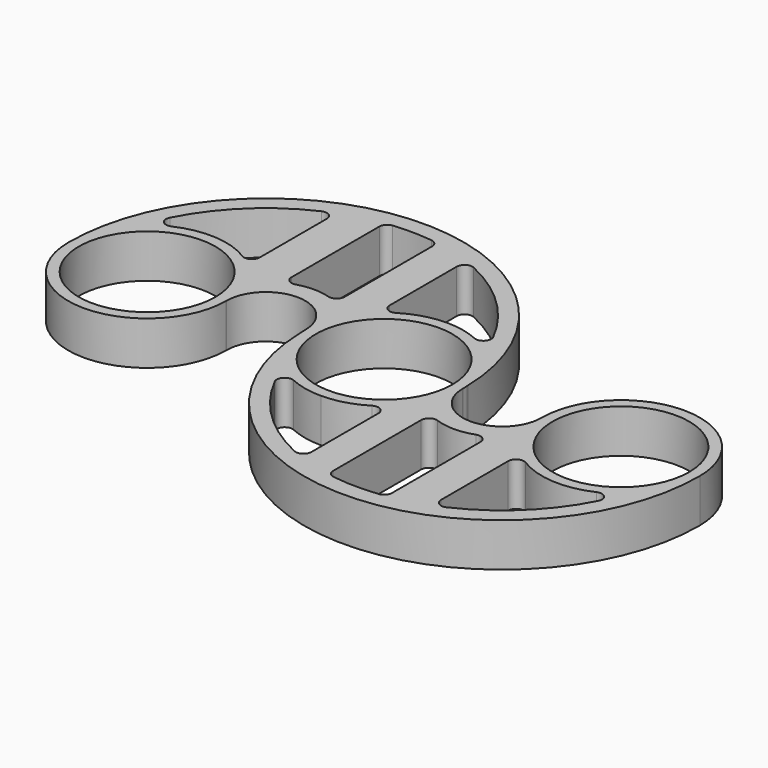
from build123d import *

# Parameters (mm, degrees)
F0_R        = 10.9855
F0_R_2      = 10.989999991
F1_DEPTH    = 7
F2_T1_DEPTH = 7
F2_T3_DEPTH = 7.1579854221
F2_T5_DEPTH = 7.1579856015
F2_T7_DEPTH = 7.1579856772
F3_R        = 1.27


# Not quite as in the source:
# - a fillet or chamfer that OpenCascade refuses, or shapes differently, is made with other operations: its cross-section is extruded or revolved along the edge and cut away or added
# - a feature names something its author has since deleted; it is built from what else it names


with BuildPart() as f1:
    # F0 (on Top) → F1 (new body)
    with BuildSketch(Plane.XY):
        with BuildLine():
            ThreePointArc((0.0122500747, -12.699994092), (8.9845861326, -8.9759240207), (12.7, 0))
            ThreePointArc((12.7, 0), (11.6341942626, 5.0926931834), (8.6156655339, 9.3306113095))
            ThreePointArc((8.6156655339, 9.3306113095), (4.6312435718, 11.8254633304), (0.0122500747, 12.699994092))
            ThreePointArc((0.0122500747, 12.699994092), (-4.6067434223, 11.8254633304), (-8.5911653844, 9.3306113095))
            ThreePointArc((-8.5911653844, 9.3306113095), (-11.6096941131, 5.0926931834), (-12.6754998505, 0))
            ThreePointArc((-12.6754998505, 0), (-11.6096941131, -5.0926931834), (-8.5911653844, -9.3306113095))
            ThreePointArc((-8.5911653844, -9.3306113095), (-4.6067434223, -11.8254633304), (0.0122500747, -12.699994092))
        make_face()
        with Locations((0.0245001495, 0)):
            Circle(F0_R, mode=Mode.SUBTRACT)
        with BuildLine():
            ThreePointArc((12.7245001495, 0), (12.716207726, 0.4588668575), (12.6913412845, 0.9171344838))
            ThreePointArc((12.6913412845, 0.9171344838), (12.6989837582, 0.4585985212), (12.7, 0))
            ThreePointArc((12.7, 0), (8.9845861326, -8.9759240207), (0.0122500747, -12.699994092))
            ThreePointArc((0.0122500747, -12.699994092), (4.6443350463, -11.8299250009), (8.6401656833, -9.3306113095))
            ThreePointArc((8.6401656833, -9.3306113095), (10.2086695664, -7.5876671836), (11.4300151579, -5.586074417))
            ThreePointArc((11.4300151579, -5.586074417), (12.3868415398, -2.9090402797), (12.7242073512, -0.086237983))
            ThreePointArc((12.7242073512, -0.086237983), (12.7242070748, -0.0431184935), (12.7245001495, 0))
        make_face()
        with BuildLine():
            ThreePointArc((25.4002735579, -0.086237983), (19.0622404546, -6.4027075191), (12.7242073512, -0.086237983))
            ThreePointArc((12.7242073512, -0.086237983), (12.3868415398, -2.9090402797), (11.4300151579, -5.586074417))
            ThreePointArc((11.4300151579, -5.586074417), (12.5867658694, -6.9038365057), (13.9769937331, -7.9724035921))
            ThreePointArc((13.9769937331, -7.9724035921), (18.7426985376, -9.3370960194), (23.5084033421, -7.9724035921))
            ThreePointArc((23.5084033421, -7.9724035921), (25.1435205419, -6.6655071902), (26.4326717576, -5.0163632895))
            ThreePointArc((26.4326717576, -5.0163632895), (25.6695984826, -2.6029975888), (25.4002735579, -0.086237983))
        make_face()
        with BuildLine():
            ThreePointArc((46.7156462935, -9.3306113095), (49.7341750222, -5.0926931834), (50.7999807596, 0))
            ThreePointArc((50.7999807596, 0), (38.0999807596, 12.7), (25.3999807596, 0))
            ThreePointArc((25.3999807596, 0), (25.4002738343, -0.0431184935), (25.4002735579, -0.086237983))
            ThreePointArc((25.4002735579, -0.086237983), (25.6695984826, -2.6029975888), (26.4326717576, -5.0163632895))
            ThreePointArc((26.4326717576, -5.0163632895), (27.7316179187, -7.3339656394), (29.4843152258, -9.3306113095))
            ThreePointArc((29.4843152258, -9.3306113095), (38.0999807596, -12.7), (46.7156462935, -9.3306113095))
        make_face()
        with Locations((38.0999807596, 0)):
            Circle(F0_R_2, mode=Mode.SUBTRACT)
        with BuildLine():
            ThreePointArc((-8.5801649897, -9.3632669913), (-11.43210855, -5.5314459322), (-12.666841135, -0.9171344838))
            ThreePointArc((-12.666841135, -0.9171344838), (19.5208281328, -31.8937955885), (50.7999807596, 0))
            ThreePointArc((50.7999807596, 0), (49.7341750222, -5.0926931834), (46.7156462935, -9.3306113095))
            ThreePointArc((46.7156462935, -9.3306113095), (40.1099512813, -20.2359805679), (29.4843152258, -27.2828340268))
            ThreePointArc((29.4843152258, -27.2828340268), (26.5384433366, -28.2337157759), (23.5084033421, -28.8671152702))
            ThreePointArc((23.5084033421, -28.8671152702), (18.7383474141, -29.2061036376), (13.9769937331, -28.7612915499))
            ThreePointArc((13.9769937331, -28.7612915499), (11.2734206382, -28.1489774328), (8.6401656833, -27.2828340268))
            ThreePointArc((8.6401656833, -27.2828340268), (-1.9735358373, -20.2484070502), (-8.5801649897, -9.3632669913))
        make_face()
        with BuildLine():
            ThreePointArc((-11.4055150084, 5.586074417), (-12.3623413903, 2.9090402797), (-12.6997072018, 0.086237983))
            ThreePointArc((-12.6997072018, 0.086237983), (-12.6997069253, 0.0431184935), (-12.7, 0))
            ThreePointArc((-12.7, 0), (-12.6917075765, -0.4588668575), (-12.666841135, -0.9171344838))
            ThreePointArc((-12.666841135, -0.9171344838), (-12.6744836087, -0.4585985212), (-12.6754998505, 0))
            ThreePointArc((-12.6754998505, 0), (-11.6096941131, 5.0926931834), (-8.5911653844, 9.3306113095))
            Line((-8.5911653844, 9.3306113095), (-8.5911653844, 9.3531747198))
            ThreePointArc((-8.5911653844, 9.3531747198), (-10.1742109205, 7.6010152049), (-11.4055150084, 5.586074417))
        make_face()
        with BuildLine():
            ThreePointArc((-22.9900462212, 8.2591606127), (-24.9149898439, 6.8653148973), (-26.4081716081, 5.0163632895))
            ThreePointArc((-26.4081716081, 5.0163632895), (-25.6450983331, 2.6029975888), (-25.3757734084, 0.086237983))
            ThreePointArc((-25.3757734084, 0.086237983), (-19.0377403051, 6.4027075191), (-12.6997072018, 0.086237983))
            ThreePointArc((-12.6997072018, 0.086237983), (-12.3623413903, 2.9090402797), (-11.4055150084, 5.586074417))
            ThreePointArc((-11.4055150084, 5.586074417), (-12.773731355, 7.0957580254), (-14.446350555, 8.2591606127))
            ThreePointArc((-14.446350555, 8.2591606127), (-18.7181983881, 9.3370960194), (-22.9900462212, 8.2591606127))
        make_face()
        with BuildLine():
            ThreePointArc((-25.3757734084, 0.086237983), (-25.6450983331, 2.6029975888), (-26.4081716081, 5.0163632895))
            ThreePointArc((-26.4081716081, 5.0163632895), (-27.7071177693, 7.3339656394), (-29.4598150763, 9.3306113095))
            ThreePointArc((-29.4598150763, 9.3306113095), (-38.0754806101, 12.7), (-46.691146144, 9.3306113095))
            ThreePointArc((-46.691146144, 9.3306113095), (-49.7096748727, 5.0926931834), (-50.7754806101, 0))
            ThreePointArc((-50.7754806101, 0), (-38.0754806101, -12.7), (-25.3754806101, 0))
            ThreePointArc((-25.3754806101, 0), (-25.3757736848, 0.0431184935), (-25.3757734084, 0.086237983))
        make_face()
        with Locations((-38.0754806101, 0)):
            Circle(F0_R_2, mode=Mode.SUBTRACT)
        with BuildLine():
            ThreePointArc((-8.5911653844, -9.3306113095), (-8.5856700083, -9.3469407745), (-8.5801649897, -9.3632669913))
            ThreePointArc((-8.5801649897, -9.3632669913), (-4.5973610293, -11.8386769348), (0.0122500747, -12.699994092))
            ThreePointArc((0.0122500747, -12.699994092), (-4.6067434223, -11.8254633304), (-8.5911653844, -9.3306113095))
        make_face()
        with BuildLine():
            ThreePointArc((-12.6754998505, 0), (-12.6744836087, -0.4585985212), (-12.666841135, -0.9171344838))
            ThreePointArc((-12.666841135, -0.9171344838), (-11.43210855, -5.5314459322), (-8.5801649897, -9.3632669913))
            ThreePointArc((-8.5801649897, -9.3632669913), (-8.5856700083, -9.3469407745), (-8.5911653844, -9.3306113095))
            ThreePointArc((-8.5911653844, -9.3306113095), (-11.6096941131, -5.0926931834), (-12.6754998505, 0))
        make_face()
        with BuildLine():
            ThreePointArc((12.7, 0), (12.6989837582, 0.4585985212), (12.6913412845, 0.9171344838))
            ThreePointArc((12.6913412845, 0.9171344838), (11.4566086995, 5.5314459323), (8.6046651392, 9.3632669913))
            ThreePointArc((8.6046651392, 9.3632669913), (8.6101701578, 9.3469407745), (8.6156655339, 9.3306113095))
            ThreePointArc((8.6156655339, 9.3306113095), (11.6341942626, 5.0926931834), (12.7, 0))
        make_face()
        with BuildLine():
            ThreePointArc((8.6156655339, 9.3306113095), (8.6101701578, 9.3469407745), (8.6046651392, 9.3632669913))
            ThreePointArc((8.6046651392, 9.3632669913), (4.6218611788, 11.8386769348), (0.0122500747, 12.699994092))
            ThreePointArc((0.0122500747, 12.699994092), (4.6312435718, 11.8254633304), (8.6156655339, 9.3306113095))
        make_face()
        with BuildLine():
            ThreePointArc((-50.7754806101, 0), (-49.7096748727, 5.0926931834), (-46.691146144, 9.3306113095))
            ThreePointArc((-46.691146144, 9.3306113095), (-40.0854511318, 20.2359805679), (-29.4598150763, 27.2828340268))
            ThreePointArc((-29.4598150763, 27.2828340268), (-26.2724748955, 28.2966277505), (-22.9900462212, 28.9389494304))
            ThreePointArc((-22.9900462212, 28.9389494304), (-18.7147163655, 29.2061132739), (-14.446350555, 28.8443464952))
            ThreePointArc((-14.446350555, 28.8443464952), (-11.4778445606, 28.2113948339), (-8.5911653844, 27.2734508175))
            ThreePointArc((-8.5911653844, 27.2734508175), (2.0071231414, 20.238946653), (8.6046651392, 9.3632669913))
            ThreePointArc((8.6046651392, 9.3632669913), (11.4566086995, 5.5314459323), (12.6913412845, 0.9171344838))
            ThreePointArc((12.6913412845, 0.9171344838), (-19.4963279834, 31.8937955885), (-50.7754806101, 0))
        make_face()
        with BuildLine():
            Line((-14.446350555, 28.8443464952), (-14.446350555, 8.2591606127))
            ThreePointArc((-14.446350555, 8.2591606127), (-12.773731355, 7.0957580254), (-11.4055150084, 5.586074417))
            ThreePointArc((-11.4055150084, 5.586074417), (-10.1742109205, 7.6010152049), (-8.5911653844, 9.3531747198))
            Line((-8.5911653844, 9.3531747198), (-8.5911653844, 27.2734508175))
            ThreePointArc((-8.5911653844, 27.2734508175), (-11.4778445606, 28.2113948339), (-14.446350555, 28.8443464952))
        make_face()
        with BuildLine():
            ThreePointArc((-29.4598150763, 9.3306113095), (-27.7071177693, 7.3339656394), (-26.4081716081, 5.0163632895))
            ThreePointArc((-26.4081716081, 5.0163632895), (-24.9149898439, 6.8653148973), (-22.9900462212, 8.2591606127))
            Line((-22.9900462212, 8.2591606127), (-22.9900462212, 28.9389494304))
            ThreePointArc((-22.9900462212, 28.9389494304), (-26.2724748955, 28.2966277505), (-29.4598150763, 27.2828340268))
            Line((-29.4598150763, 27.2828340268), (-29.4598150763, 9.3306113095))
        make_face()
        with BuildLine():
            Line((8.6401656833, -9.3306113095), (8.6401656833, -27.2828340268))
            ThreePointArc((8.6401656833, -27.2828340268), (11.2734206382, -28.1489774328), (13.9769937331, -28.7612915499))
            Line((13.9769937331, -28.7612915499), (13.9769937331, -7.9724035921))
            ThreePointArc((13.9769937331, -7.9724035921), (12.5867658694, -6.9038365057), (11.4300151579, -5.586074417))
            ThreePointArc((11.4300151579, -5.586074417), (10.2086695664, -7.5876671836), (8.6401656833, -9.3306113095))
        make_face()
        with BuildLine():
            Line((29.4843152258, -27.2828340268), (29.4843152258, -9.3306113095))
            ThreePointArc((29.4843152258, -9.3306113095), (27.7316179187, -7.3339656394), (26.4326717576, -5.0163632895))
            ThreePointArc((26.4326717576, -5.0163632895), (25.1435205419, -6.6655071902), (23.5084033421, -7.9724035921))
            Line((23.5084033421, -7.9724035921), (23.5084033421, -28.8671152702))
            ThreePointArc((23.5084033421, -28.8671152702), (26.5384433366, -28.2337157759), (29.4843152258, -27.2828340268))
        make_face()
    extrude(amount=F1_DEPTH)

    # F2: fillet of radius 5.08 on 9 edges, made by hand

    # F2_s2 → F2_t1 (join)
    with BuildSketch(Plane.XY):
        with BuildLine():
            ThreePointArc((-50.7755312412, 0.0104518732), (-50.7754943345, 0.0004688293), (-50.7754770463, -0.0095142678))
            ThreePointArc((-50.7754770463, -0.0095142678), (-50.7754797192, -0.0047571342), (-50.7754806101, 0))
            ThreePointArc((-50.7754806101, 0), (-50.7755063559, 0.0052259345), (-50.7755312412, 0.0104518732))
        make_face()
        with BuildLine():
            ThreePointArc((-12.6731476592, -0.8254261976), (-12.6677935321, -0.9217143052), (-12.6642681854, -1.018086699))
            ThreePointArc((-12.6642681854, -1.018086699), (-12.6655948117, -0.9676116147), (-12.666841135, -0.9171344838))
            ThreePointArc((-12.666841135, -0.9171344838), (-12.6700773725, -0.8712860467), (-12.6731476592, -0.8254261976))
        make_face()
        with BuildLine():
            ThreePointArc((12.6976478087, 0.8254261976), (12.6922936816, 0.9217143052), (12.6887683349, 1.018086699))
            ThreePointArc((12.6887683349, 1.018086699), (12.6900949612, 0.9676116147), (12.6913412845, 0.9171344838))
            ThreePointArc((12.6913412845, 0.9171344838), (12.694577522, 0.8712860467), (12.6976478087, 0.8254261976))
        make_face()
        with BuildLine():
            ThreePointArc((50.8000313907, -0.0104518732), (50.799994484, -0.0004688294), (50.7999771958, 0.0095142678))
            ThreePointArc((50.7999771958, 0.0095142678), (50.7999798687, 0.0047571342), (50.7999807596, 0))
            ThreePointArc((50.7999807596, 0), (50.8000065054, -0.0052259345), (50.8000313907, -0.0104518732))
        make_face()
    extrude(amount=F2_T1_DEPTH)

    # F2_s4 → F2_t3 (cut)
    with BuildSketch(Plane.XY.offset(-0.0789927111)):
        with BuildLine():
            ThreePointArc((-12.6998402645, 0.0182342924), (-12.6999615812, -0.0066812361), (-12.6999606939, -0.03159706))
            ThreePointArc((-12.6999606939, -0.03159706), (-12.6999901735, -0.0157985422), (-12.7, 0))
            ThreePointArc((-12.7, 0), (-12.6999135747, 0.0091170887), (-12.6998402645, 0.0182342924))
        make_face()
    extrude(amount=F2_T3_DEPTH, mode=Mode.SUBTRACT)

    # F2_s6 → F2_t5 (cut)
    with BuildSketch(Plane.XY.offset(-0.0789928007)):
        with BuildLine():
            ThreePointArc((-25.3756403458, 0.0182342804), (-25.375519029, -0.0066812601), (-25.3755199164, -0.0315970958))
            ThreePointArc((-25.3755199164, -0.0315970958), (-25.3754904367, -0.0157985601), (-25.3754806101, 0))
            ThreePointArc((-25.3754806101, 0), (-25.3755670356, 0.0091170828), (-25.3756403458, 0.0182342804))
        make_face()
        with BuildLine():
            ThreePointArc((25.4000200658, 0.0315970958), (25.4000191785, 0.0066812601), (25.4001404953, -0.0182342804))
            ThreePointArc((25.4001404953, -0.0182342804), (25.4000671851, -0.0091170828), (25.3999807596, 0))
            ThreePointArc((25.3999807596, 0), (25.3999905862, 0.0157985601), (25.4000200658, 0.0315970958))
        make_face()
    extrude(amount=F2_T5_DEPTH, mode=Mode.SUBTRACT)

    # F2_s8 → F2_t7 (cut)
    with BuildSketch(Plane.XY.offset(-0.0789928386)):
        with BuildLine():
            ThreePointArc((12.7243404138, -0.0182342754), (12.7244617306, 0.0066812701), (12.7244608432, 0.031597111))
            ThreePointArc((12.7244608432, 0.031597111), (12.7244903229, 0.0157985677), (12.7245001495, 0))
            ThreePointArc((12.7245001495, 0), (12.724413724, -0.0091170802), (12.7243404138, -0.0182342754))
        make_face()
    extrude(amount=F2_T7_DEPTH, mode=Mode.SUBTRACT)

    # F3
    f3_edges = [f1.edges().sort_by_distance(p)[0] for p in [
        (29.484315, -27.282834, 3.5),
        (29.484315, -9.330611, 3.5),
        (46.715646, -9.330611, 3.5),
        (23.508403, -7.972404, 3.5),
        (13.976994, -7.972404, 3.5),
        (23.508403, -28.867115, 3.5),
        (13.976994, -28.761292, 3.5),
        (8.640166, -27.282834, 3.5),
        (8.640166, -9.330611, 3.5),
        (-8.580165, -9.363267, 3.5),
        (-22.990046, 28.938949, 3.5),
        (-8.591165, 27.273451, 3.5),
        (8.604665, 9.363267, 3.5),
        (-8.591165, 9.330611, 3.5),
        (-22.990046, 8.259161, 3.5),
        (-14.446351, 8.259161, 3.5),
        (-14.446351, 28.844346, 3.5),
        (-29.459815, 9.330611, 3.5),
        (-29.459815, 27.282834, 3.5),
        (-46.691146, 9.330611, 3.5),
    ]]
    fillet(f3_edges, radius=F3_R)


solid = f1.part
